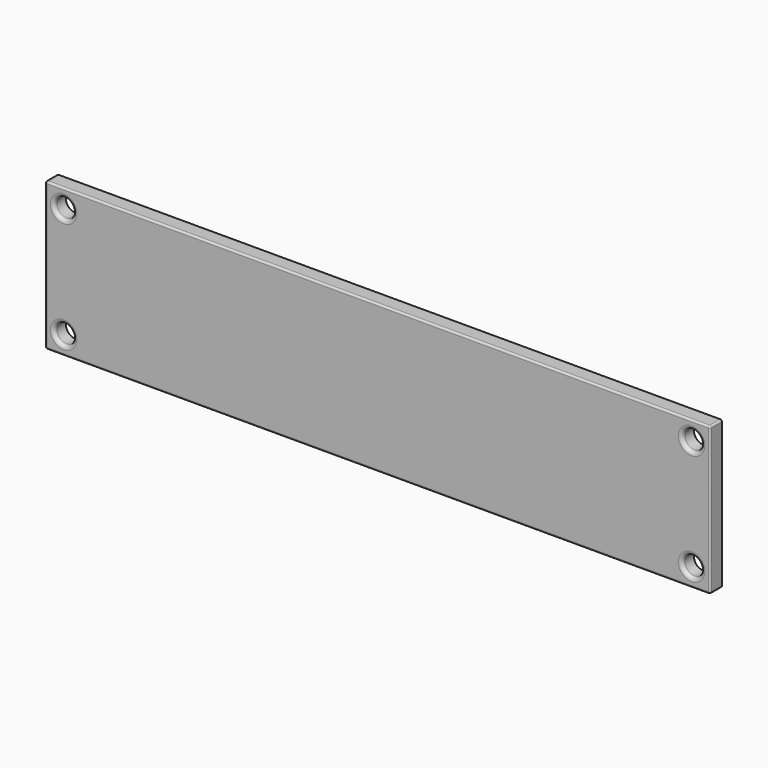
from build123d import *

# Parameters (mm, degrees)
F0_W         = 180
F0_H         = 40
F0_R         = 2.5751263091
F1_DEPTH     = 4
F2_R         = 1
F3_R         = 0.5
F4_TEXT_SIZE = 7.4830462234
F5_DEPTH     = 1


# Not quite as in the source:
# - a feature names something its author has since deleted; it is built from what else it names
# - Text() gives the source's letters only with a copy of the font that has no kerning and outlines rounded to 1/6400 em; it was checked with that copy


with BuildPart() as f1:
    # F0 (on Front) → F1 (new body)
    with BuildSketch(Plane.XZ):
        Rectangle(F0_W, F0_H)
        with Locations((-85, -15)):
            Circle(F0_R, mode=Mode.SUBTRACT)
        with Locations((85, -15)):
            Circle(F0_R, mode=Mode.SUBTRACT)
        with Locations((-85, 15)):
            Circle(F0_R, mode=Mode.SUBTRACT)
        with Locations((85, 15)):
            Circle(F0_R, mode=Mode.SUBTRACT)
    extrude(amount=F1_DEPTH)

    # F2
    f2_edges = [f1.edges().sort_by_distance(p)[0] for p in [
        (-87.575126, -4, 15),
        (-87.575126, -4, -15),
        (82.424874, -4, 15),
        (82.424874, -4, -15),
    ]]
    fillet(f2_edges, radius=F2_R)

    # F3
    f3_edges = [f1.edges().sort_by_distance(p)[0] for p in [
        (0, -4, 20),
        (-90, -4, 0),
        (0, -4, -20),
        (90, -4, 0),
        (-90, -2, 20),
        (-90, -2, -20),
        (90, -2, 20),
        (90, -2, -20),
    ]]
    fillet(f3_edges, radius=F3_R)

    # F4 (on face) → F5 (join)
    with BuildSketch(Plane(origin=(0, 0, 0), x_dir=(-1, 0, 0), z_dir=(0, 1, 0))):
        with Locations((-70.5961091444, -2.6410444846)):
            Text('Berea Cigar Body', F4_TEXT_SIZE, font='Open Sans', text_align=(TextAlign.LEFT, TextAlign.BOTTOM))
    extrude(amount=F5_DEPTH)

    # F6: F1 across plane


with BuildPart() as f1_1:
    add(f1.part)
    add(f1.part.mirror(Plane.YZ))


solid = f1_1.part
